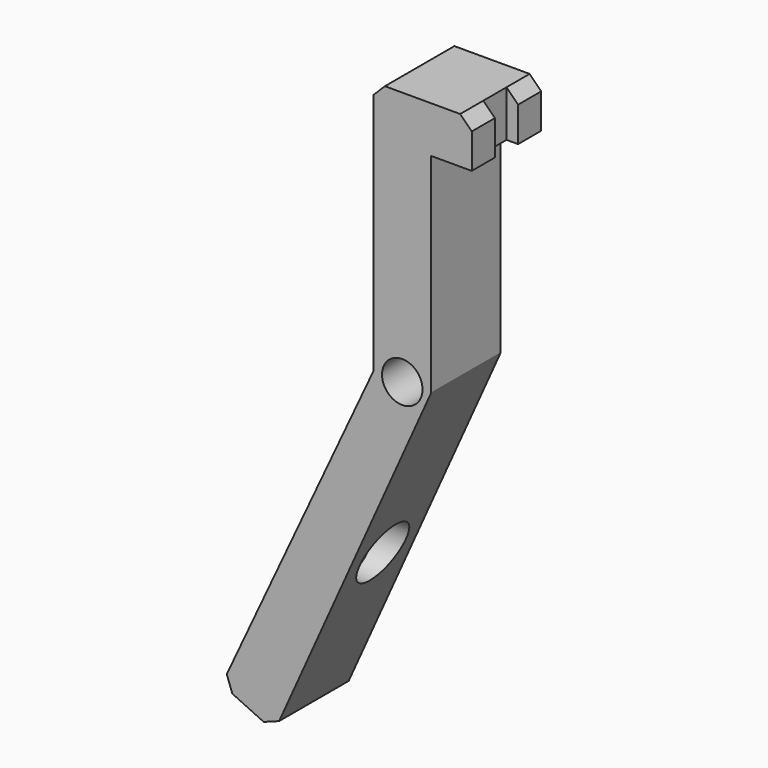
from build123d import *

# Parameters (mm, degrees)
F0_R        = 1.75
F1_DEPTH    = 7.5
F2_T1_DEPTH = 12.6433659759
F2_T3_DEPTH = 12.7137209508
F3_R        = 2.5
F4_DEPTH    = 5
F5_W        = 2.5
F5_H        = 3
F6_DEPTH    = 1
F7_W        = 1
F7_H        = 2.5
F8_DEPTH    = 25


# Not quite as in the source:
# - a fillet or chamfer that OpenCascade refuses, or shapes differently, is made with other operations: its cross-section is extruded or revolved along the edge and cut away or added


with BuildPart() as f1:
    # F0 (on Front) → F1 (new body)
    with BuildSketch(Plane.XZ):
        Polygon((-29.1562567131, -15.4619954874), (-25.6562567131, -15.4619954874), (-25.6562567131, -11.4619954874), (-34.1562567131, -11.4619954874), (-34.1562567131, -33.4619954874), (-47.2335256009, -61.5062891187), (-42.7019866657, -63.6193804274), (-29.1562567131, -33.4619954874), align=None)
        with Locations((-31.6562567131, -33.4619954874)):
            Circle(F0_R, mode=Mode.SUBTRACT)
    extrude(amount=F1_DEPTH)

    # F2: chamfer of 1 on 4 edges, made by hand

    # F2_s2 → F2_t1 (cut)
    with BuildSketch(Plane.XZ.offset(-2.571682988)):
        Polygon((-33.1562567131, -11.4619954874), (-34.1562567131, -12.4619954874), (-34.1562567131, -11.4619954874), align=None)
        Polygon((-25.6562567131, -12.4619954874), (-26.6562567131, -11.4619954874), (-25.6562567131, -11.4619954874), align=None)
        Polygon((-46.8109073392, -60.5999813317), (-46.3272178139, -61.9289073804), (-47.2335256009, -61.5062891187), align=None)
    extrude(amount=F2_T1_DEPTH, mode=Mode.SUBTRACT)

    # F2_s4 → F2_t3 (cut)
    with BuildSketch(Plane.XZ.offset(-2.6068604754)):
        Polygon((-42.2864056117, -62.6941561786), (-43.6212292029, -63.1907305926), (-42.7019866657, -63.6193804274), align=None)
    extrude(amount=F2_T3_DEPTH, mode=Mode.SUBTRACT)

    # F3 (on face) → F4 (cut)
    with BuildSketch(Plane(origin=(-34.1562567131, 0, 0), x_dir=(0, -1, 0), z_dir=(-1, 0, 0))):
        with Locations((3.75, -49.4619954874)):
            Circle(F3_R)
    extrude(amount=F4_DEPTH, mode=Mode.SUBTRACT)

    # F5 (on face) → F6 (cut)
    with BuildSketch(Plane.YZ.offset(-25.6562567131)):
        with Locations((-3.75, -13.9619954874)):
            Rectangle(F5_W, F5_H)
    extrude(amount=-F6_DEPTH, mode=Mode.SUBTRACT)

    # F7 (on face) → F8 (cut)
    with BuildSketch(Plane(origin=(0, 0, -12.4619954874), x_dir=(1, 0, 0), z_dir=(0, 0, -1))):
        with Locations((-26.1562567131, 3.75)):
            Rectangle(F7_W, F7_H)
    extrude(amount=-F8_DEPTH, mode=Mode.SUBTRACT)


solid = f1.part
